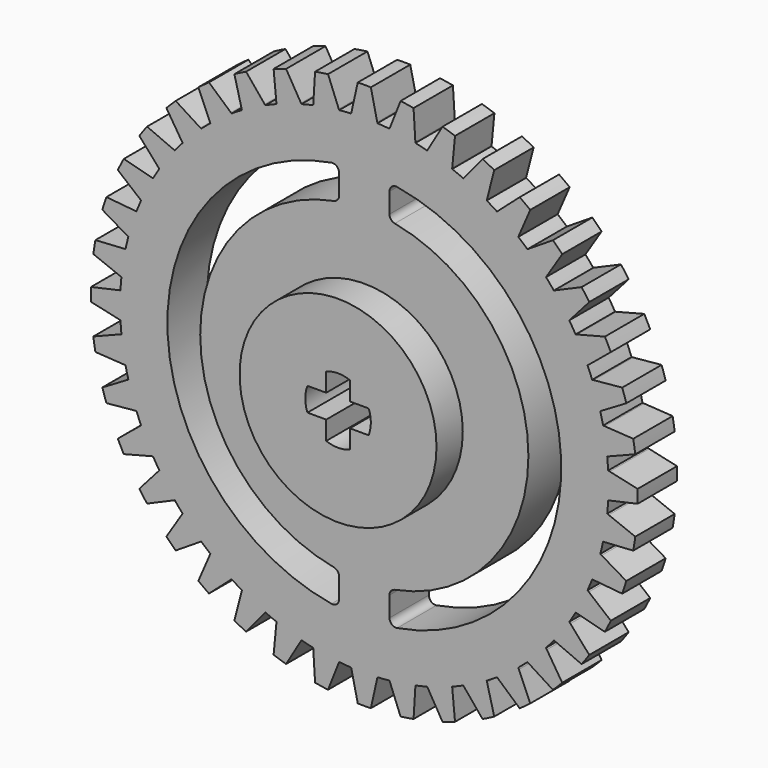
from build123d import *

# Parameters (mm, degrees)
F0_R     = 7.5
F1_DEPTH = 1.875
F3_COUNT = 40
F4_DEPTH = 4.375
F6_DEPTH = 8.751
F9_DEPTH = 6.251


with BuildPart() as f1:
    # F0 (on Front) → F1 (new body, symmetric)
    with BuildSketch(Plane.XZ):
        with BuildLine():
            Line((0.9846328973, 18.6421247134), (0.5, 20.8189967338))
            ThreePointArc((0.5, 20.8189967338), (0, 20.825), (-0.5, 20.8189967338))
            Line((-0.5, 20.8189967338), (-0.973161251, 18.6936530064))
            Line((-0.973161251, 18.6936530064), (-1, 18.573098826))
            ThreePointArc((-1, 18.573098826), (0, 18.6), (1, 18.573098826))
            Line((1, 18.573098826), (0.9846328973, 18.6421247134))
        make_face()
        with BuildLine():
            ThreePointArc((18.6, 0), (13.5011110654, 12.7937484734), (1, 18.573098826))
            ThreePointArc((1, 18.573098826), (0, 18.6), (-1, 18.573098826))
            ThreePointArc((-1, 18.573098826), (-12.7937484734, -13.5011110654), (18.6, 0))
        make_face()
        Circle(F0_R, mode=Mode.SUBTRACT)
    extrude(amount=F1_DEPTH, both=True)


with BuildPart() as f3_1:
    # F3: instance of F1
    add(f1.part.rotate(Axis((0, -1.875, 0), (0, -1, 0)), 1 * 360 / F3_COUNT))


with BuildPart() as f3_2:
    # F3: instance of F1
    add(f1.part.rotate(Axis((0, -1.875, 0), (0, -1, 0)), 2 * 360 / F3_COUNT))


with BuildPart() as f3_3:
    # F3: instance of F1
    add(f1.part.rotate(Axis((0, -1.875, 0), (0, -1, 0)), 3 * 360 / F3_COUNT))


with BuildPart() as f3_4:
    # F3: instance of F1
    add(f1.part.rotate(Axis((0, -1.875, 0), (0, -1, 0)), 4 * 360 / F3_COUNT))


with BuildPart() as f3_5:
    # F3: instance of F1
    add(f1.part.rotate(Axis((0, -1.875, 0), (0, -1, 0)), 5 * 360 / F3_COUNT))


with BuildPart() as f3_6:
    # F3: instance of F1
    add(f1.part.rotate(Axis((0, -1.875, 0), (0, -1, 0)), 6 * 360 / F3_COUNT))


with BuildPart() as f3_7:
    # F3: instance of F1
    add(f1.part.rotate(Axis((0, -1.875, 0), (0, -1, 0)), 7 * 360 / F3_COUNT))


with BuildPart() as f3_8:
    # F3: instance of F1
    add(f1.part.rotate(Axis((0, -1.875, 0), (0, -1, 0)), 8 * 360 / F3_COUNT))


with BuildPart() as f3_9:
    # F3: instance of F1
    add(f1.part.rotate(Axis((0, -1.875, 0), (0, -1, 0)), 9 * 360 / F3_COUNT))


with BuildPart() as f3_10:
    # F3: instance of F1
    add(f1.part.rotate(Axis((0, -1.875, 0), (0, -1, 0)), 10 * 360 / F3_COUNT))


with BuildPart() as f3_11:
    # F3: instance of F1
    add(f1.part.rotate(Axis((0, -1.875, 0), (0, -1, 0)), 11 * 360 / F3_COUNT))


with BuildPart() as f3_12:
    # F3: instance of F1
    add(f1.part.rotate(Axis((0, -1.875, 0), (0, -1, 0)), 12 * 360 / F3_COUNT))


with BuildPart() as f3_13:
    # F3: instance of F1
    add(f1.part.rotate(Axis((0, -1.875, 0), (0, -1, 0)), 13 * 360 / F3_COUNT))


with BuildPart() as f3_14:
    # F3: instance of F1
    add(f1.part.rotate(Axis((0, -1.875, 0), (0, -1, 0)), 14 * 360 / F3_COUNT))


with BuildPart() as f3_15:
    # F3: instance of F1
    add(f1.part.rotate(Axis((0, -1.875, 0), (0, -1, 0)), 15 * 360 / F3_COUNT))


with BuildPart() as f3_16:
    # F3: instance of F1
    add(f1.part.rotate(Axis((0, -1.875, 0), (0, -1, 0)), 16 * 360 / F3_COUNT))


with BuildPart() as f3_17:
    # F3: instance of F1
    add(f1.part.rotate(Axis((0, -1.875, 0), (0, -1, 0)), 17 * 360 / F3_COUNT))


with BuildPart() as f3_18:
    # F3: instance of F1
    add(f1.part.rotate(Axis((0, -1.875, 0), (0, -1, 0)), 18 * 360 / F3_COUNT))


with BuildPart() as f3_19:
    # F3: instance of F1
    add(f1.part.rotate(Axis((0, -1.875, 0), (0, -1, 0)), 19 * 360 / F3_COUNT))


with BuildPart() as f3_20:
    # F3: instance of F1
    add(f1.part.rotate(Axis((0, -1.875, 0), (0, -1, 0)), 20 * 360 / F3_COUNT))


with BuildPart() as f3_21:
    # F3: instance of F1
    add(f1.part.rotate(Axis((0, -1.875, 0), (0, -1, 0)), 21 * 360 / F3_COUNT))


with BuildPart() as f3_22:
    # F3: instance of F1
    add(f1.part.rotate(Axis((0, -1.875, 0), (0, -1, 0)), 22 * 360 / F3_COUNT))


with BuildPart() as f3_23:
    # F3: instance of F1
    add(f1.part.rotate(Axis((0, -1.875, 0), (0, -1, 0)), 23 * 360 / F3_COUNT))


with BuildPart() as f3_24:
    # F3: instance of F1
    add(f1.part.rotate(Axis((0, -1.875, 0), (0, -1, 0)), 24 * 360 / F3_COUNT))


with BuildPart() as f3_25:
    # F3: instance of F1
    add(f1.part.rotate(Axis((0, -1.875, 0), (0, -1, 0)), 25 * 360 / F3_COUNT))


with BuildPart() as f3_26:
    # F3: instance of F1
    add(f1.part.rotate(Axis((0, -1.875, 0), (0, -1, 0)), 26 * 360 / F3_COUNT))


with BuildPart() as f3_27:
    # F3: instance of F1
    add(f1.part.rotate(Axis((0, -1.875, 0), (0, -1, 0)), 27 * 360 / F3_COUNT))


with BuildPart() as f3_28:
    # F3: instance of F1
    add(f1.part.rotate(Axis((0, -1.875, 0), (0, -1, 0)), 28 * 360 / F3_COUNT))


with BuildPart() as f3_29:
    # F3: instance of F1
    add(f1.part.rotate(Axis((0, -1.875, 0), (0, -1, 0)), 29 * 360 / F3_COUNT))


with BuildPart() as f3_30:
    # F3: instance of F1
    add(f1.part.rotate(Axis((0, -1.875, 0), (0, -1, 0)), 30 * 360 / F3_COUNT))


with BuildPart() as f3_31:
    # F3: instance of F1
    add(f1.part.rotate(Axis((0, -1.875, 0), (0, -1, 0)), 31 * 360 / F3_COUNT))


with BuildPart() as f3_32:
    # F3: instance of F1
    add(f1.part.rotate(Axis((0, -1.875, 0), (0, -1, 0)), 32 * 360 / F3_COUNT))


with BuildPart() as f3_33:
    # F3: instance of F1
    add(f1.part.rotate(Axis((0, -1.875, 0), (0, -1, 0)), 33 * 360 / F3_COUNT))


with BuildPart() as f3_34:
    # F3: instance of F1
    add(f1.part.rotate(Axis((0, -1.875, 0), (0, -1, 0)), 34 * 360 / F3_COUNT))


with BuildPart() as f3_35:
    # F3: instance of F1
    add(f1.part.rotate(Axis((0, -1.875, 0), (0, -1, 0)), 35 * 360 / F3_COUNT))


with BuildPart() as f3_36:
    # F3: instance of F1
    add(f1.part.rotate(Axis((0, -1.875, 0), (0, -1, 0)), 36 * 360 / F3_COUNT))


with BuildPart() as f3_37:
    # F3: instance of F1
    add(f1.part.rotate(Axis((0, -1.875, 0), (0, -1, 0)), 37 * 360 / F3_COUNT))


with BuildPart() as f3_38:
    # F3: instance of F1
    add(f1.part.rotate(Axis((0, -1.875, 0), (0, -1, 0)), 38 * 360 / F3_COUNT))


with BuildPart() as f3_39:
    # F3: instance of F1
    add(f1.part.rotate(Axis((0, -1.875, 0), (0, -1, 0)), 39 * 360 / F3_COUNT))


with BuildPart() as f1_1:
    add(f1.part)

    add(f3_1.part)  # F4 merges F3_1

    add(f3_2.part)  # F4 merges F3_2

    add(f3_3.part)  # F4 merges F3_3

    add(f3_4.part)  # F4 merges F3_4

    add(f3_5.part)  # F4 merges F3_5

    add(f3_6.part)  # F4 merges F3_6

    add(f3_7.part)  # F4 merges F3_7

    add(f3_8.part)  # F4 merges F3_8

    add(f3_9.part)  # F4 merges F3_9

    add(f3_10.part)  # F4 merges F3_10

    add(f3_11.part)  # F4 merges F3_11

    add(f3_12.part)  # F4 merges F3_12

    add(f3_13.part)  # F4 merges F3_13

    add(f3_14.part)  # F4 merges F3_14

    add(f3_15.part)  # F4 merges F3_15

    add(f3_16.part)  # F4 merges F3_16

    add(f3_17.part)  # F4 merges F3_17

    add(f3_18.part)  # F4 merges F3_18

    add(f3_19.part)  # F4 merges F3_19

    add(f3_20.part)  # F4 merges F3_20

    add(f3_21.part)  # F4 merges F3_21

    add(f3_22.part)  # F4 merges F3_22

    add(f3_23.part)  # F4 merges F3_23

    add(f3_24.part)  # F4 merges F3_24

    add(f3_25.part)  # F4 merges F3_25

    add(f3_26.part)  # F4 merges F3_26

    add(f3_27.part)  # F4 merges F3_27

    add(f3_28.part)  # F4 merges F3_28

    add(f3_29.part)  # F4 merges F3_29

    add(f3_30.part)  # F4 merges F3_30

    add(f3_31.part)  # F4 merges F3_31

    add(f3_32.part)  # F4 merges F3_32

    add(f3_33.part)  # F4 merges F3_33

    add(f3_34.part)  # F4 merges F3_34

    add(f3_35.part)  # F4 merges F3_35

    add(f3_36.part)  # F4 merges F3_36

    add(f3_37.part)  # F4 merges F3_37

    add(f3_38.part)  # F4 merges F3_38

    add(f3_39.part)  # F4 merges F3_39
    # F0 (on Front) → F4 (join, symmetric)
    with BuildSketch(Plane.XZ):
        Circle(F0_R)
    extrude(amount=F4_DEPTH, both=True)

    # F5 (on face) → F6 (cut, through all)
    with BuildSketch(Plane.XZ.offset(4.375)):
        with BuildLine():
            ThreePointArc((2.3313088598, -0.9), (2.4567195445, -0.4577445572), (2.499, 0))
            ThreePointArc((2.499, 0), (2.4567195445, 0.4577445572), (2.3313088598, 0.9))
            Line((2.3313088598, 0.9), (0.9, 0.9))
            Line((0.9, 0.9), (0.9, 2.3313088598))
            ThreePointArc((0.9, 2.3313088598), (0, 2.499), (-0.9, 2.3313088598))
            Line((-0.9, 2.3313088598), (-0.9, 0.9))
            Line((-0.9, 0.9), (-2.3313088598, 0.9))
            ThreePointArc((-2.3313088598, 0.9), (-2.499, 0), (-2.3313088598, -0.9))
            Line((-2.3313088598, -0.9), (-0.9, -0.9))
            Line((-0.9, -0.9), (-0.9, -2.3313088598))
            ThreePointArc((-0.9, -2.3313088598), (0, -2.499), (0.9, -2.3313088598))
            Line((0.9, -2.3313088598), (0.9, -0.9))
            Line((0.9, -0.9), (2.3313088598, -0.9))
        make_face()
    extrude(amount=-F6_DEPTH, mode=Mode.SUBTRACT)

    # F7: union 

    # F8 (on face) → F9 (cut, through all)
    with BuildSketch(Plane.XZ.offset(1.875)):
        with BuildLine():
            ThreePointArc((-1.9177844384, 14.2970038263), (-2.0950507545, 14.6788977505), (-2.5011563156, 14.7900039583))
            ThreePointArc((-2.5011563156, 14.7900039583), (-15, 0), (-2.5011563156, -14.7900039583))
            ThreePointArc((-2.5011563156, -14.7900039583), (-2.0950507545, -14.6788977505), (-1.9177844384, -14.2970038263))
            Line((-1.9177844384, -14.2970038263), (-1.9177844384, -12.7731874804))
            ThreePointArc((-1.9177844384, -12.7731874804), (-2.0327546638, -12.4542014733), (-2.3247927292, -12.2819110388))
            ThreePointArc((-2.3247927292, -12.2819110388), (-12.5, 0), (-2.3247927292, 12.2819110388))
            ThreePointArc((-2.3247927292, 12.2819110388), (-2.0327546638, 12.4542014733), (-1.9177844384, 12.7731874804))
            Line((-1.9177844384, 12.7731874804), (-1.9177844384, 14.2970038263))
        make_face()
        with BuildLine():
            Line((1.9177844384, -12.7731874804), (1.9177844384, -14.2970038263))
            ThreePointArc((1.9177844384, -14.2970038263), (2.0950507545, -14.6788977505), (2.5011563156, -14.7900039583))
            ThreePointArc((2.5011563156, -14.7900039583), (15, 0), (2.5011563156, 14.7900039583))
            ThreePointArc((2.5011563156, 14.7900039583), (2.0950507545, 14.6788977505), (1.9177844384, 14.2970038263))
            Line((1.9177844384, 14.2970038263), (1.9177844384, 12.7731874804))
            ThreePointArc((1.9177844384, 12.7731874804), (2.0327546638, 12.4542014733), (2.3247927292, 12.2819110388))
            ThreePointArc((2.3247927292, 12.2819110388), (12.5, 0), (2.3247927292, -12.2819110388))
            ThreePointArc((2.3247927292, -12.2819110388), (2.0327546638, -12.4542014733), (1.9177844384, -12.7731874804))
        make_face()
    extrude(amount=-F9_DEPTH, mode=Mode.SUBTRACT)


solid = f1_1.part
